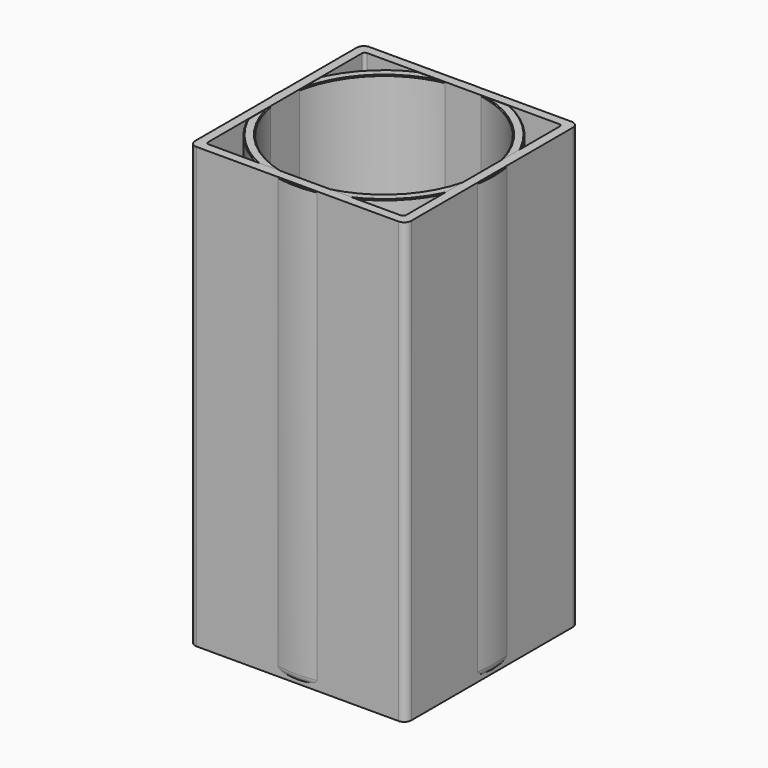
from build123d import *

# Parameters (mm, degrees)
F3_SIZE   = 0.635
F4_R      = 6
F5_DEPTH  = 5
F5_TAPER  = 4
F6_R      = 1
F8_DEPTH  = 305
F9_W      = 137.2
F9_H      = 137.2
F10_DEPTH = 13


with BuildPart() as f2:
    # F0 (on Front) → F2 (revolve)
    with BuildSketch(Plane.XZ):
        with BuildLine():
            Line((-69.85, 0), (-43.27, 0))
            ThreePointArc((-43.27, 0), (-42.3719743879, 0.3719743879), (-42, 1.27))
            Line((-42, 1.27), (-42, 11.43))
            ThreePointArc((-42, 11.43), (-42.3719743879, 12.3280256121), (-43.27, 12.7))
            Line((-43.27, 12.7), (-68.58, 12.7))
            ThreePointArc((-68.58, 12.7), (-69.4780256121, 13.0719743879), (-69.85, 13.97))
            Line((-69.85, 13.97), (-69.85, 304.8))
            Line((-69.85, 304.8), (-76.2, 304.8))
            Line((-76.2, 304.8), (-76.2, 6.35))
            ThreePointArc((-76.2, 6.35), (-74.3401280605, 1.8598719395), (-69.85, 0))
        make_face()
    revolve(axis=Axis((0, 0, 44.2740730941), (0, 0, 1)))

    # F3
    f3_edges = [f2.edges().sort_by_distance(p)[0] for p in [
        (69.85, 0, 304.8),
        (76.2, 0, 304.8),
    ]]
    chamfer(f3_edges, length=F3_SIZE)

    # F4 (on face) → F5 (join)
    with BuildSketch(Plane(origin=(0, 0, 0), x_dir=(1, 0, 0), z_dir=(0, 0, -1))):
        with Locations((0, 59)):
            Circle(F4_R)
        with Locations((-59, 0)):
            Circle(F4_R)
        with Locations((0, -59)):
            Circle(F4_R)
        with Locations((59, 0)):
            Circle(F4_R)
    extrude(amount=F5_DEPTH, taper=F5_TAPER)

    # F6
    f6_edges = [f2.edges().sort_by_distance(p)[0] for p in [
        (-5.650366, -59, -5),
        (-64.650366, 0, -5),
        (-5.650366, 59, -5),
        (53.349634, 0, -5),
    ]]
    fillet(f6_edges, radius=F6_R)


with BuildPart() as f8:
    # F7 (on Top) → F8 (new body)
    with BuildSketch(Plane.XY):
        with BuildLine():
            Line((-70, -75), (70, -75))
            ThreePointArc((70, -75), (73.5355339059, -73.5355339059), (75, -70))
            Line((75, -70), (75, 70))
            ThreePointArc((75, 70), (73.5355339059, 73.5355339059), (70, 75))
            Line((70, 75), (-70, 75))
            ThreePointArc((-70, 75), (-73.5355339059, 73.5355339059), (-75, 70))
            Line((-75, 70), (-75, -70))
            ThreePointArc((-75, -70), (-73.5355339059, -73.5355339059), (-70, -75))
        make_face()
        with BuildLine():
            Line((68.6, 66.6), (68.6, -66.6))
            ThreePointArc((68.6, -66.6), (68.0142135624, -68.0142135624), (66.6, -68.6))
            Line((66.6, -68.6), (-66.6, -68.6))
            ThreePointArc((-66.6, -68.6), (-68.0142135624, -68.0142135624), (-68.6, -66.6))
            Line((-68.6, -66.6), (-68.6, 66.6))
            ThreePointArc((-68.6, 66.6), (-68.0142135624, 68.0142135624), (-66.6, 68.6))
            Line((-66.6, 68.6), (66.6, 68.6))
            ThreePointArc((66.6, 68.6), (68.0142135624, 68.0142135624), (68.6, 66.6))
        make_face(mode=Mode.SUBTRACT)
    extrude(amount=F8_DEPTH)

    # F9 (on face) → F10 (join)
    with BuildSketch(Plane(origin=(0, 0, 0), x_dir=(1, 0, 0), z_dir=(0, 0, -1))):
        Rectangle(F9_W, F9_H)
    extrude(amount=-F10_DEPTH)


solid = Compound([f2.part, f8.part])
